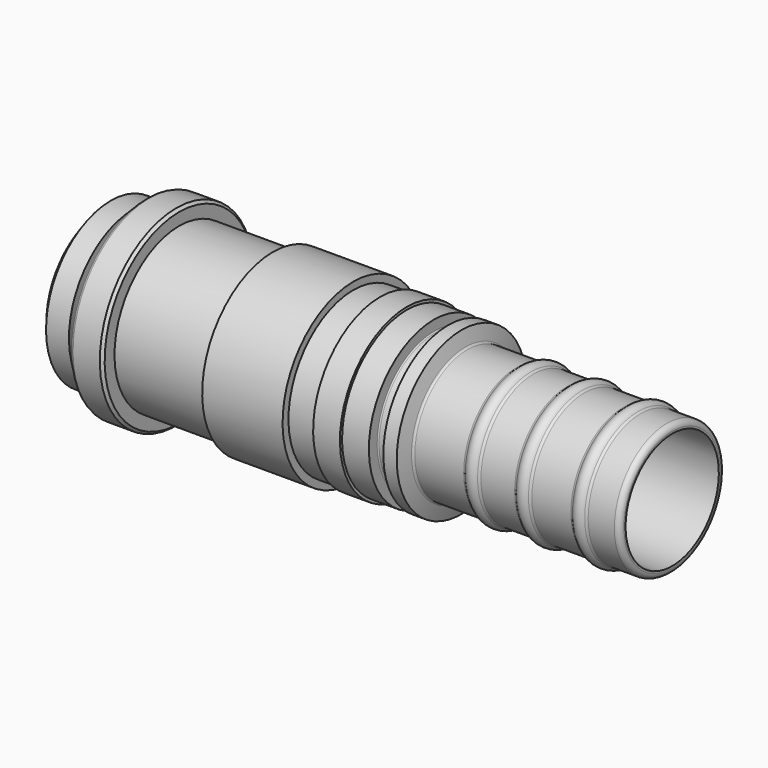
from build123d import *

# Parameters (mm, degrees)
F2_R = 1.2
F3_R = 2
F4_R = 0.8
F5_R = 0.4


# Not quite as in the source:
# - a fillet or chamfer that OpenCascade refuses, or shapes differently, is made with other operations: its cross-section is extruded or revolved along the edge and cut away or added


with BuildPart() as f1:
    # F0 (on Front) → F1 (revolve)
    with BuildSketch(Plane.XZ):
        with BuildLine():
            Line((0, 21.75), (213, 21.75))
            Line((213, 21.75), (213, 24.5))
            Line((213, 24.5), (200.5980762114, 24.5))
            ThreePointArc((200.5980762114, 24.5), (198, 26), (195.4019237886, 24.5))
            Line((195.4019237886, 24.5), (179.5980762114, 24.5))
            ThreePointArc((179.5980762114, 24.5), (177, 26), (174.4019237886, 24.5))
            Line((174.4019237886, 24.5), (160.5980762114, 24.5))
            ThreePointArc((160.5980762114, 24.5), (158, 26), (155.4019237886, 24.5))
            Line((155.4019237886, 24.5), (135.9407078565, 24.5))
            Line((135.9407078565, 24.5), (134.4, 30.25))
            Line((134.4, 30.25), (129.4, 30.25))
            Line((129.4, 30.25), (129.4, 26))
            Line((129.4, 26), (124, 26))
            Line((124, 26), (124, 30.25))
            Line((124, 30.25), (114, 30.25))
            Line((114, 30.25), (114, 31.25))
            Line((114, 31.25), (104, 31.25))
            Line((104, 31.25), (104, 30.25))
            Line((104, 30.25), (94, 30.25))
            Line((94, 30.25), (94, 33))
            Line((94, 33), (64, 33))
            Line((64, 33), (64, 30.15))
            Line((64, 30.15), (29, 30.15))
            Line((29, 30.15), (29, 35.75))
            Line((29, 35.75), (17.6, 35.75))
            Line((17.6, 35.75), (12, 30.15))
            Line((12, 30.15), (3.4529714459, 30.15))
            Line((3.4529714459, 30.15), (0, 25.65))
            Line((0, 25.65), (0, 21.75))
        make_face()
    revolve(axis=Axis((44.485598996, 0, 0), (1, 0, 0)))

    # F2
    f2_edges = [f1.edges().sort_by_distance(p)[0] for p in [
        (200.598076, 0, -24.5),
        (179.598076, 0, -24.5),
        (160.598076, 0, -24.5),
        (155.401924, 0, -24.5),
        (174.401924, 0, -24.5),
        (195.401924, 0, -24.5),
    ]]
    fillet(f2_edges, radius=F2_R)

    # F3
    f3_edges = [f1.edges().sort_by_distance(p)[0] for p in [
        (213, 0, -24.5),
    ]]
    fillet(f3_edges, radius=F3_R)

    # F4
    f4_edges = [f1.edges().sort_by_distance(p)[0] for p in [
        (135.940708, 0, -24.5),
    ]]
    fillet(f4_edges, radius=F4_R)

    # F5
    f5_edges = [f1.edges().sort_by_distance(p)[0] for p in [
        (124, 0, -26),
        (129.4, 0, -26),
    ]]
    fillet(f5_edges, radius=F5_R)

    # F6: chamfer of 1 on 4 edges, made by hand

    # F6_s1 → F6_t2 (revolve, cut)
    with BuildSketch(Plane.XZ):
        Polygon((29, 34.75), (28, 35.75), (29, 35.75), align=None)
    revolve(axis=Axis((29, 0, 0), (1, 0, 0)), mode=Mode.SUBTRACT)

    # F6_s3 → F6_t4 (revolve, cut)
    with BuildSketch(Plane.XZ):
        Polygon((18.0142135624, 35.75), (17.3071067812, 35.4571067812), (17.6, 35.75), align=None)
    revolve(axis=Axis((17.6, 0, 0), (1, 0, 0)), mode=Mode.SUBTRACT)

    # F6_s5 → F6_t6 (revolve, cut)
    with BuildSketch(Plane.XZ):
        Polygon((0.2066466597, 25.9193071701), (0, 25.3105457411), (0, 25.65), align=None)
    revolve(axis=Axis((0, 0, 0), (1, 0, 0)), mode=Mode.SUBTRACT)

    # F6_s7 → F6_t8 (revolve, cut)
    with BuildSketch(Plane.XZ):
        Polygon((0, 22.75), (1, 21.75), (0, 21.75), align=None)
    revolve(axis=Axis((0, 0, 0), (1, 0, 0)), mode=Mode.SUBTRACT)


solid = f1.part
